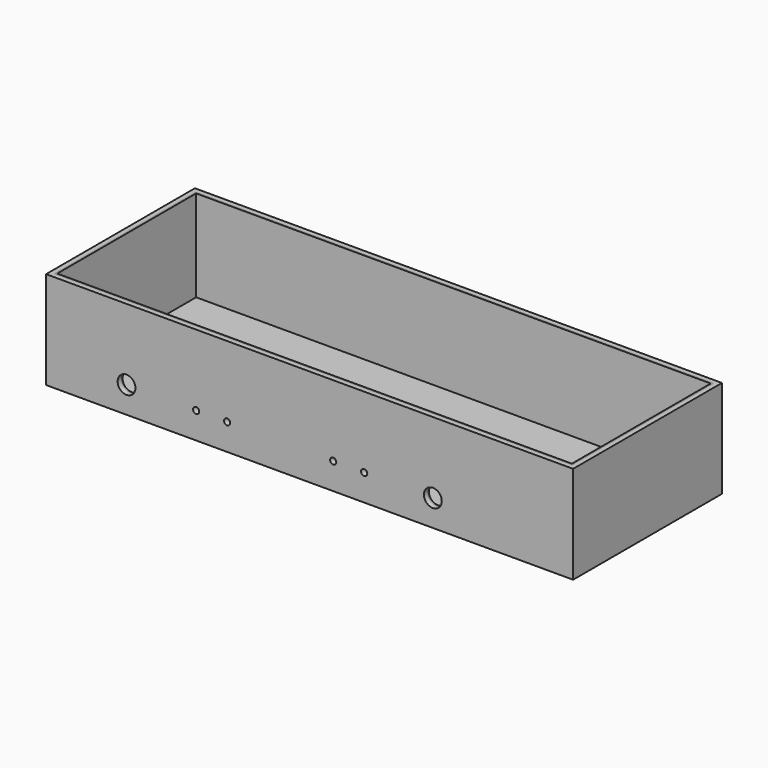
from build123d import *

# Parameters (mm, degrees)
F0_W     = 850
F0_H     = 300
F1_DEPTH = 7.5
F2_W     = 850
F2_H     = 300
F2_W_2   = 835
F2_H_2   = 285
F3_DEPTH = 150
F4_DEPTH = 2.5
F5_W     = 835
F5_H     = 285
F5_W_2   = 830
F5_H_2   = 280
F6_DEPTH = 147.5
F7_R     = 5
F7_R_2   = 14.39
F8_DEPTH = 25


with BuildPart() as f1:
    # F0 (on Top) → F1 (new body)
    with BuildSketch(Plane.XY):
        Rectangle(F0_W, F0_H)
    extrude(amount=F1_DEPTH)

    # F2 (on face) → F3 (join)
    with BuildSketch(Plane.XY.offset(7.5)):
        Rectangle(F2_W, F2_H)
        Rectangle(F2_W_2, F2_H_2, mode=Mode.SUBTRACT)
    extrude(amount=F3_DEPTH)


with BuildPart() as f4:
    # F4 (new): a face of the model
    f4_faces = [f1.part.faces().sort_by_distance(p)[0] for p in [
        (0, 0, 7.5),
    ]]
    extrude(f4_faces, amount=F4_DEPTH)

    # F5 (on face) → F6 (join)
    with BuildSketch(Plane.XY.offset(10)):
        Rectangle(F5_W, F5_H)
        Rectangle(F5_W_2, F5_H_2, mode=Mode.SUBTRACT)
    extrude(amount=F6_DEPTH)


with BuildPart() as f8_tool:
    # F7 (on face) → F8 (new body)
    with BuildSketch(Plane.XZ.offset(150)):
        with Locations((-133, 42.655)):
            Circle(F7_R)
        with Locations((38, 42.655)):
            Circle(F7_R)
        with Locations((88, 42.655)):
            Circle(F7_R)
        with Locations((-183, 42.655)):
            Circle(F7_R)
        with Locations((198.78, 42.655)):
            Circle(F7_R_2)
        with Locations((-295.22, 42.655)):
            Circle(F7_R_2)
    extrude(amount=-F8_DEPTH)


with BuildPart() as f1_1:
    add(f1.part)

    # F8: cut by f8_tool
    add(f8_tool.part, mode=Mode.SUBTRACT)


with BuildPart() as f4_1:
    add(f4.part)

    # F8: cut by f8_tool
    add(f8_tool.part, mode=Mode.SUBTRACT)


solid = Compound([f1_1.part, f4_1.part])
